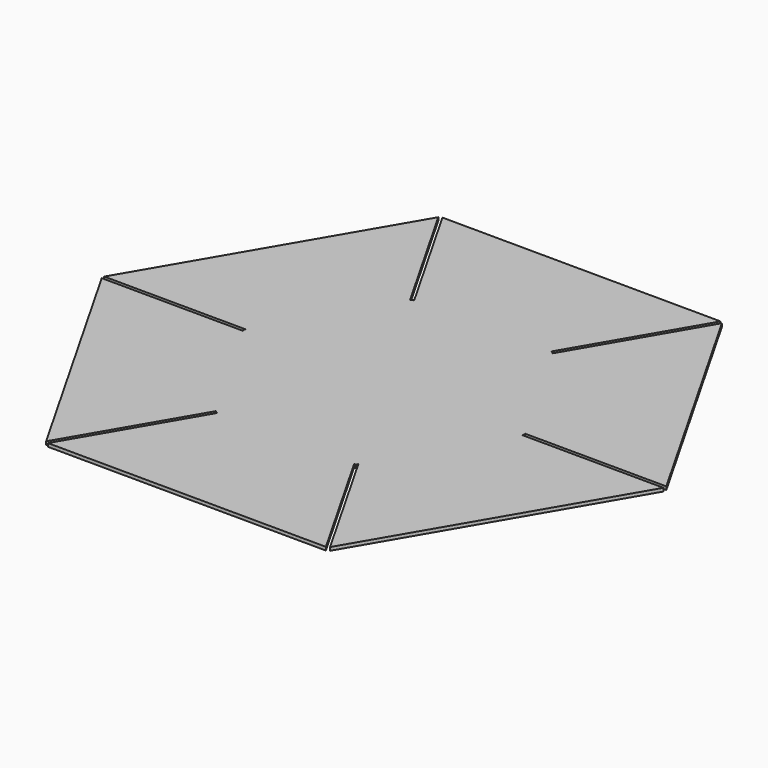
from build123d import *

# Parameters (mm, degrees)
F1_DEPTH = 1.5


# Not quite as in the source:
# - ends of sketch curves that miss each other by under 0.0002 mm in the source are joined


with BuildPart() as f1:
    # F0 (on Top) → F1 (new body)
    with BuildSketch(Plane.XY):
        Polygon((-154.7862010079, -56.3197720771), (-155.698514, -56.31515), (-156.1119683507, -57.0229680515), (-188.1119961072, -0.943063637), (-252.2166275849, -110.6877438524), (-187.6499915883, -111.0148592346), (-188.0469170019, -111.6943803821), (-187.578521744, -112.5152405744), (-252.1451579752, -112.188125191), (-189.1969680657, -222.5045451407), (-156.6379224358, -166.7385013741), (-156.261298, -167.398534), (-155.2892116972, -167.4034589083), (-187.8405636484, -223.1563251995), (-60.9469641109, -223.7992090591), (-92.9469916323, -167.7193050566), (-92.127277, -167.723458), (-91.6671171884, -166.9356819838), (-59.667332984, -223.0151595742), (4.3105823215, -113.4874126049), (-60.2555620411, -113.1602997135), (-59.778874, -112.344228), (-60.1688938721, -111.6607195518), (4.3977421328, -111.987834934), (-58.5385800691, -1.6922148149), (-90.9212471101, -57.156163237), (-91.0976251965, -57.4582577209), (-91.4381361233, -56.861513861), (-91.8289476292, -56.638734186), (-92.3545377772, -56.6360713738), (-59.8031858283, -0.8832050865), (-186.7862285296, -0.239868074), (-155.0159777331, -55.9170894017), align=None)
        Polygon((-124.7326106109, -112.0151510591), (-124.6877867318, -112.0153781513), (-124.7103900886, -112.0540924243), align=None, mode=Mode.SUBTRACT)
        Polygon((-123.0005820296, -112.023926074), (-122.955962742, -112.0241521297), (-122.9784629293, -112.0626896976), align=None, mode=Mode.SUBTRACT)
    extrude(amount=F1_DEPTH)


solid = f1.part
